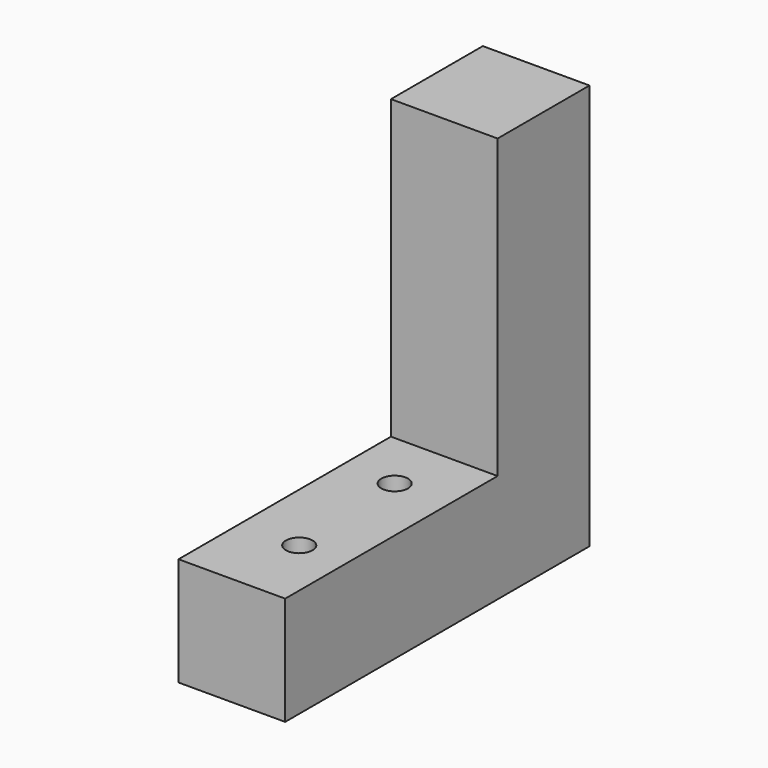
from build123d import *

# Parameters (mm, degrees)
F1_DEPTH = 25.4
F3_D     = 6.35
F5_D     = 6.35


# Not quite as in the source:
# - a feature names something its author has since deleted; it is built from what else it names


with BuildPart() as f1:
    # F0 (on Right) → F1 (new body)
    with BuildSketch(Plane.YZ):
        Polygon((14.3006006256, -31.3609689474), (-48.9231087267, -31.3609689474), (-48.9231087267, -57.2024062276), (41.6473634541, -57.2024062276), (41.6473634541, 39.3893681467), (14.3006006256, 39.3893681467), align=None)
    extrude(amount=F1_DEPTH)

    # F3 (through all)
    with Locations(Plane.XY.offset(-31.3609689474)):
        with Locations((14.0417637303, -30.5415708572)):
            Hole(F3_D / 2)

    # F5 (through all)
    with Locations(Plane.XY.offset(-31.3609689474)):
        with Locations((12.3347630724, 0)):
            Hole(F5_D / 2)


solid = f1.part
